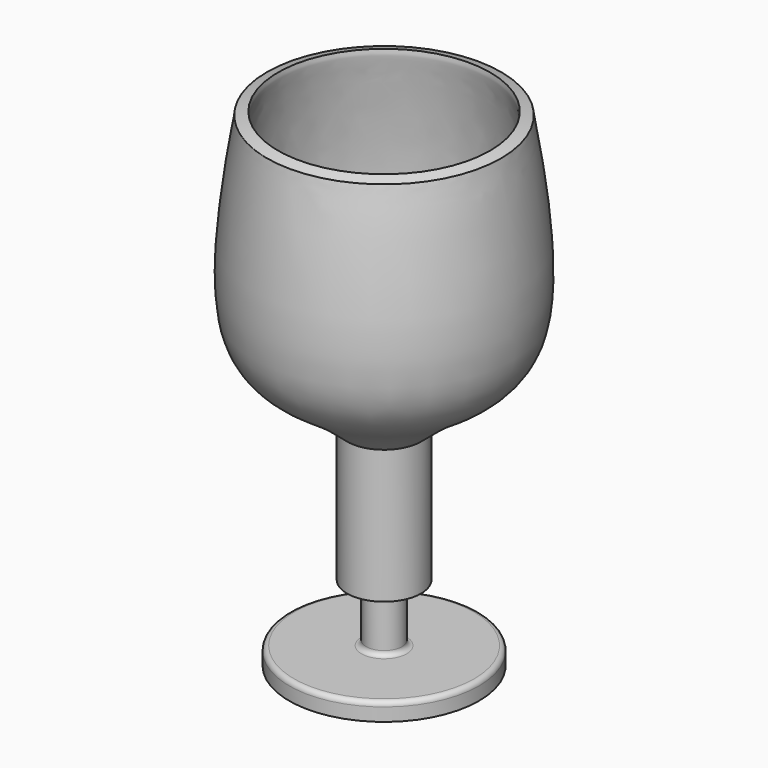
from build123d import *

# Parameters (mm, degrees)
F2_R = 0.5


# Not quite as in the source:
# - a feature of the source that left no trace in its solid (it failed there, or was rolled back) is left out
# - the dataset's text gives a spline's control points without its knots; the knots are read off the source's solid


with BuildPart() as f1:
    # F0 (on Front) → F1 (revolve)
    with BuildSketch(Plane.XZ):
        with BuildLine():
            Line((0, 8.8922893628), (0, 0))
            Line((0, 0), (10, 0))
            Line((10, 0), (10, 1.8884923775))
            Line((10, 1.8884923775), (1.8822399434, 1.8884923775))
            Line((1.8822399434, 1.8884923775), (1.8822399434, 7.9723326489))
            Line((1.8822399434, 7.9723326489), (3.9016692663, 7.9723326489))
            Line((3.9016692663, 7.9723326489), (3.9016692663, 22.0649164012))
            add(Edge.make_bspline(
                [(3.9016692663, 22.0649164012), (5.1630344119, 23.1520306668), (8.0559152247, 25.6452753955), (16.5026077823, 29.9379306564), (12.263488456, 50.8664231488), (12.3197676064, 51.0582432728), (12.3233571649, 51.0704778135)],
                knots=[0, 0, 0, 0, 0.2311293716, 0.5300841921, 0.9700281494, 1, 1, 1, 1], degree=3))
            Line((12.3233571649, 51.0704778135), (11.1718934655, 51.4083120162))
            add(Edge.make_bspline(
                [(3.1182529682, 22.9739045768), (3.4593403907, 23.2678725877), (4.1477996012, 23.8612916433), (5.055986388, 24.612670911), (5.8294364602, 25.2158290825), (6.4375839903, 25.6679744102), (7.0775050494, 26.1193928261), (7.7560186195, 26.5667311764), (8.4251192748, 26.9969284999), (9.2952385489, 27.5836159192), (10.3082664571, 28.3821097797), (11.1679720476, 29.3787760328), (11.7453344155, 30.3863434128), (12.1149836837, 31.2792473003), (12.4063741535, 32.3328106346), (12.6064087785, 33.5969680598), (12.7182156401, 35.0371100675), (12.7583513738, 37.1240288557), (12.6305002665, 39.940511974), (12.3457983074, 42.7678000329), (12.0752385257, 44.8846941108), (11.8638140518, 46.3626203182), (11.656802466, 47.6938398023), (11.4987113533, 48.6504829476), (11.3872612278, 49.3063855837), (11.3127390143, 49.7393978893), (11.2487872649, 50.1095476693), (11.196769712, 50.4138822278), (11.1642496864, 50.6115467989), (11.1446042442, 50.7412492276), (11.1324663607, 50.8302814164), (11.1222249941, 50.9294704016), (11.1171182056, 51.0396395949), (11.1237031708, 51.1661769089), (11.1386792065, 51.2763017797), (11.1621810328, 51.3767208912), (11.1714256361, 51.4067174809), (11.1718934655, 51.4083120162)],
                knots=[1.1e-09, 1.1e-09, 1.1e-09, 1.1e-09, 0.0625, 0.125, 0.15625, 0.1875, 0.21875, 0.25, 0.28125, 0.3125, 0.375, 0.4375, 0.46875, 0.5, 0.53125, 0.5625, 0.59375, 0.625, 0.6875, 0.75, 0.78125, 0.8125, 0.84375, 0.875, 0.890625, 0.90625, 0.921875, 0.9375, 0.953125, 0.9609375, 0.96875, 0.9765625, 0.984375, 0.98828125, 0.9921875, 0.99609375, 1, 1, 1, 1], degree=3))
            Line((3.1182529682, 22.9739045768), (3.1182529682, 8.8922893628))
            Line((3.1182529682, 8.8922893628), (1.4163269661, 8.8922893628))
            Line((1.4163269661, 8.8922893628), (0, 8.8922893628))
        make_face()
    revolve(axis=Axis((0, 0, 4.4461446814), (0, 0, -1)))

    # F2
    f2_edges = [f1.edges().sort_by_distance(p)[0] for p in [
        (-1.88224, 0, 1.888492),
        (-1.88224, 0, 7.972333),
        (1.88224, 0, 4.930413),
        (-10, 0, 1.888492),
    ]]
    fillet(f2_edges, radius=F2_R)


solid = f1.part
